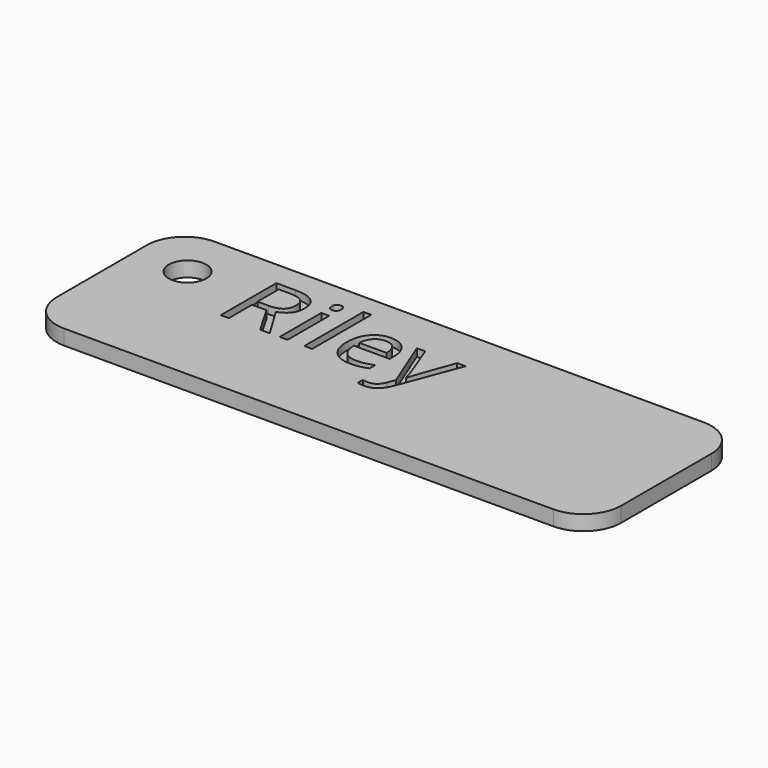
from build123d import *

# Parameters (mm, degrees)
F1_DEPTH     = 2
F3_D         = 5
F4_TEXT_SIZE = 12.9166680078
F5_DEPTH     = 1


# Not quite as in the source:
# - Text() gives the source's letters only with a copy of the font that has no kerning and outlines rounded to 1/6400 em; it was checked with that copy


with BuildPart() as f1:
    # F0 (on Top) → F1 (new body)
    with BuildSketch(Plane.XY):
        with BuildLine():
            ThreePointArc((37.5, 7.5), (36.0355339059, 11.0355339059), (32.5, 12.5))
            Line((32.5, 12.5), (-32.5, 12.5))
            ThreePointArc((-32.5, 12.5), (-36.0355339059, 11.0355339059), (-37.5, 7.5))
            Line((-37.5, 7.5), (-37.5, -7.5))
            ThreePointArc((-37.5, -7.5), (-36.0355339059, -11.0355339059), (-32.5, -12.5))
            Line((-32.5, -12.5), (32.5, -12.5))
            ThreePointArc((32.5, -12.5), (36.0355339059, -11.0355339059), (37.5, -7.5))
            Line((37.5, -7.5), (37.5, 7.5))
        make_face()
    extrude(amount=F1_DEPTH)

    # F3 (through all)
    with Locations(Plane.XY.offset(2)):
        with Locations((-30.5, 5.5)):
            Hole(F3_D / 2)

    # F4 (on face) → F5 (cut)
    with BuildSketch(Plane.XY.offset(2)):
        with Locations((-22.950001061, 0)):
            Text('Riley', F4_TEXT_SIZE, font='Open Sans', text_align=(TextAlign.LEFT, TextAlign.BOTTOM))
    extrude(amount=-F5_DEPTH, mode=Mode.SUBTRACT)


solid = f1.part
